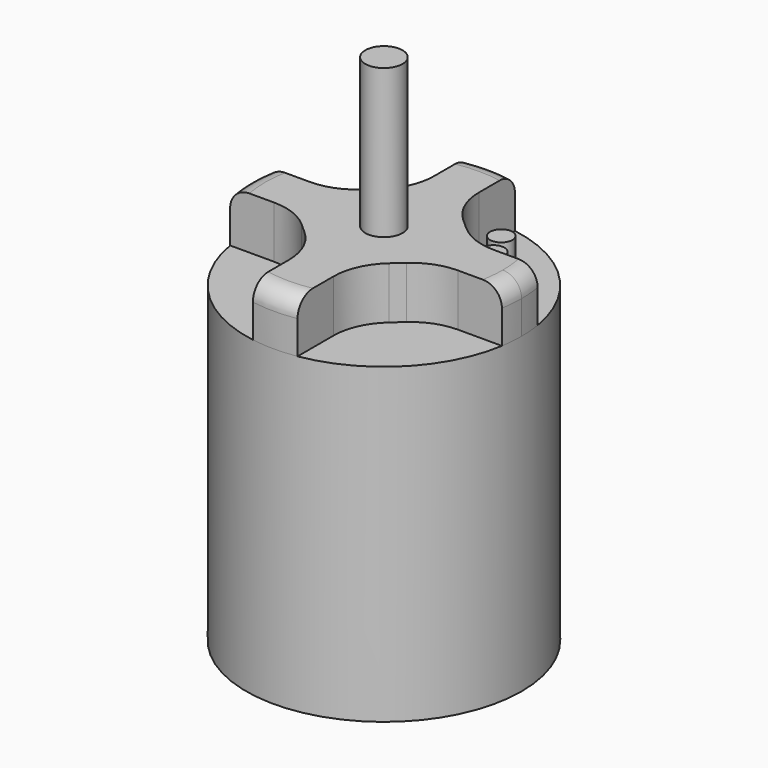
from build123d import *

# Parameters (mm, degrees)
F0_R     = 18.5
F1_DEPTH = 42
F3_DEPTH = 7
F4_R     = 2.54
F5_R     = 2.5
F6_DEPTH = 20
F8_R     = 1.5
F7_R     = 1.5
F9_DEPTH = 3


with BuildPart() as f1:
    # F0 (on Top) → F1 (new body)
    with BuildSketch(Plane.XY):
        Circle(F0_R)
    extrude(amount=F1_DEPTH)

    # F2 (on face) → F3 (join)
    with BuildSketch(Plane.XY.offset(42)):
        with BuildLine():
            ThreePointArc((-18.2551362635, 3), (-18.5, 0), (-18.2551362635, -3))
            Line((-18.2551362635, -3), (-12.357306623, -3))
            ThreePointArc((-12.357306623, -3), (-9.5173301957, -3.5232332201), (-7.0502937278, -5.0242229525))
            Line((-7.0502937278, -5.0242229525), (-5.6619374598, -6.2636447322))
            ThreePointArc((-5.6619374598, -6.2636447322), (-3.695866688, -8.9516216481), (-3, -12.2083721348))
            Line((-3, -12.2083721348), (-3, -18.2551362635))
            ThreePointArc((-3, -18.2551362635), (0, -18.5), (3, -18.2551362635))
            Line((3, -18.2551362635), (3, -12.2083721348))
            ThreePointArc((3, -12.2083721348), (3.695866688, -8.9516216481), (5.6619374598, -6.2636447322))
            Line((5.6619374598, -6.2636447322), (7.0502937278, -5.0242229525))
            ThreePointArc((7.0502937278, -5.0242229525), (9.5173301957, -3.5232332201), (12.357306623, -3))
            Line((12.357306623, -3), (18.2551362635, -3))
            ThreePointArc((18.2551362635, -3), (18.4386824485, -1.5049882267), (18.5, 0))
            ThreePointArc((18.5, 0), (18.4386824485, 1.5049882267), (18.2551362635, 3))
            Line((18.2551362635, 3), (12.357306623, 3))
            ThreePointArc((12.357306623, 3), (9.5173301957, 3.5232332201), (7.0502937278, 5.0242229525))
            Line((7.0502937278, 5.0242229525), (5.6619374598, 6.2636447322))
            ThreePointArc((5.6619374598, 6.2636447322), (3.695866688, 8.9516216481), (3, 12.2083721348))
            Line((3, 12.2083721348), (3, 18.2551362635))
            ThreePointArc((3, 18.2551362635), (0, 18.5), (-3, 18.2551362635))
            Line((-3, 18.2551362635), (-3, 12.2083721348))
            ThreePointArc((-3, 12.2083721348), (-3.695866688, 8.9516216481), (-5.6619374598, 6.2636447322))
            Line((-5.6619374598, 6.2636447322), (-7.0502937278, 5.0242229525))
            ThreePointArc((-7.0502937278, 5.0242229525), (-9.5173301957, 3.5232332201), (-12.357306623, 3))
            Line((-12.357306623, 3), (-18.2551362635, 3))
        make_face()
    extrude(amount=F3_DEPTH)

    # F4
    f4_edges = [f1.edges().sort_by_distance(p)[0] for p in [
        (0, 18.5, 49),
        (-18.5, 0, 49),
        (0, -18.5, 49),
        (18.5, 0, 49),
    ]]
    fillet(f4_edges, radius=F4_R)

    # F5 (on face) → F6 (join)
    with BuildSketch(Plane.XY.offset(49)):
        Circle(F5_R)
    extrude(amount=F6_DEPTH)

    # F8 (on face) + F7 (on face) → F9 (join)
    with BuildSketch(Plane.XY.offset(42)):
        with Locations((6.1871920723, 11.9740978757)):
            Circle(F8_R)
    with BuildSketch(Plane.XY.offset(42)):
        with Locations((7.7906422209, 8.6364694748)):
            Circle(F7_R)
        with Locations((10.0058761309, 5.7833763727)):
            Circle(F7_R)
    extrude(amount=F9_DEPTH)


solid = f1.part
